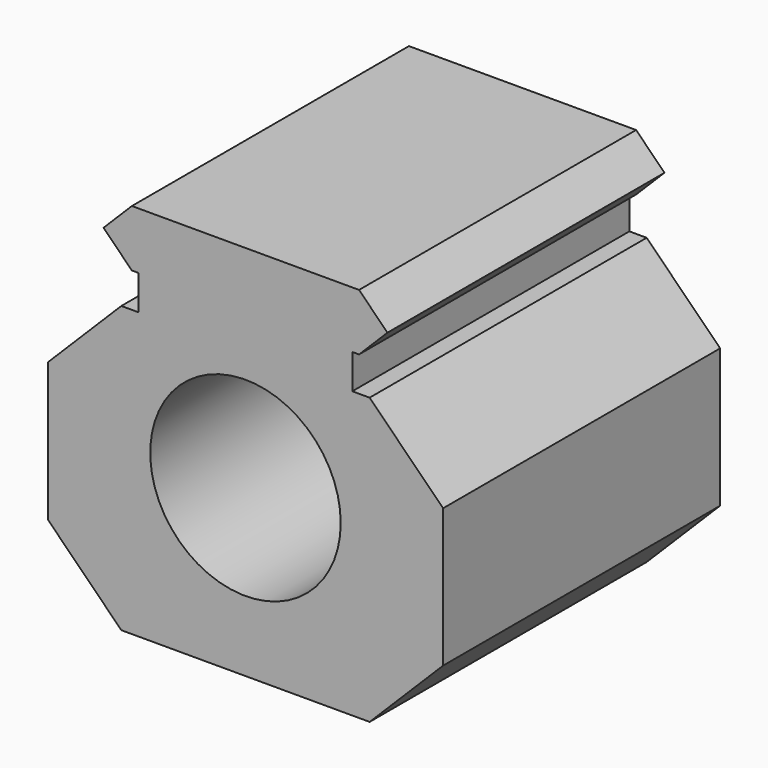
from build123d import *

# Parameters (mm, degrees)
F1_DEPTH    = 25.4
F3_D        = 13.97
F3_DEPTH    = 25.4
F3_TIP      = 4.1970114239
F4_T1_DEPTH = 37.157734621


# Not quite as in the source:
# - a fillet or chamfer that OpenCascade refuses, or shapes differently, is made with other operations: its cross-section is extruded or revolved along the edge and cut away or added


with BuildPart() as f1:
    # F0 (on Front) → F1 (new body)
    with BuildSketch(Plane.XZ):
        Polygon((10.6172, 19.1102290041), (0, 19.1102290041), (0, -8.5316783412), (9.1059, -8.5316783412), (14.4940536726, -3.1435246685), (14.4940536726, 7.0164753315), (9.1059, 12.4046290041), (7.8359, 12.4046290041), (7.8359, 14.9446290041), (10.6172, 14.9446290041), align=None)
        Polygon((0, -8.5316783412), (0, 19.1102290041), (-10.6172, 19.1102290041), (-10.6172, 14.9446290041), (-7.8359, 14.9446290041), (-7.8359, 12.4046290041), (-9.1059, 12.4046290041), (-14.4940536726, 7.0164753315), (-14.4940536726, -3.1435246685), (-9.1059, -8.5316783412), align=None)
    extrude(amount=F1_DEPTH)

    # F3
    with Locations(Plane(origin=(0, 0, 0), x_dir=(-1, 0, 0), z_dir=(0, 1, 0))):
        with Locations((0, 3.620829666)):
            Hole(F3_D / 2, depth=F3_DEPTH)
            with Locations((0, 0, -(F3_DEPTH + F3_TIP / 2))):  # 118° drill point
                Cone(0, F3_D / 2, F3_TIP, mode=Mode.SUBTRACT)

    # F4: chamfer of 2.286 on 4 edges, made by hand

    # F4_s2 → F4_t1 (cut)
    with BuildSketch(Plane.XZ.offset(-5.8788673105)):
        Polygon((8.3312, 14.9446290041), (10.6172, 17.2306290041), (10.6172, 14.9446290041), align=None)
        Polygon((10.6172, 16.8242290041), (8.3312, 19.1102290041), (10.6172, 19.1102290041), align=None)
        Polygon((-8.3312, 19.1102290041), (-10.6172, 16.8242290041), (-10.6172, 19.1102290041), align=None)
        Polygon((-10.6172, 17.2306290041), (-8.3312, 14.9446290041), (-10.6172, 14.9446290041), align=None)
    extrude(amount=F4_T1_DEPTH, mode=Mode.SUBTRACT)


solid = f1.part
